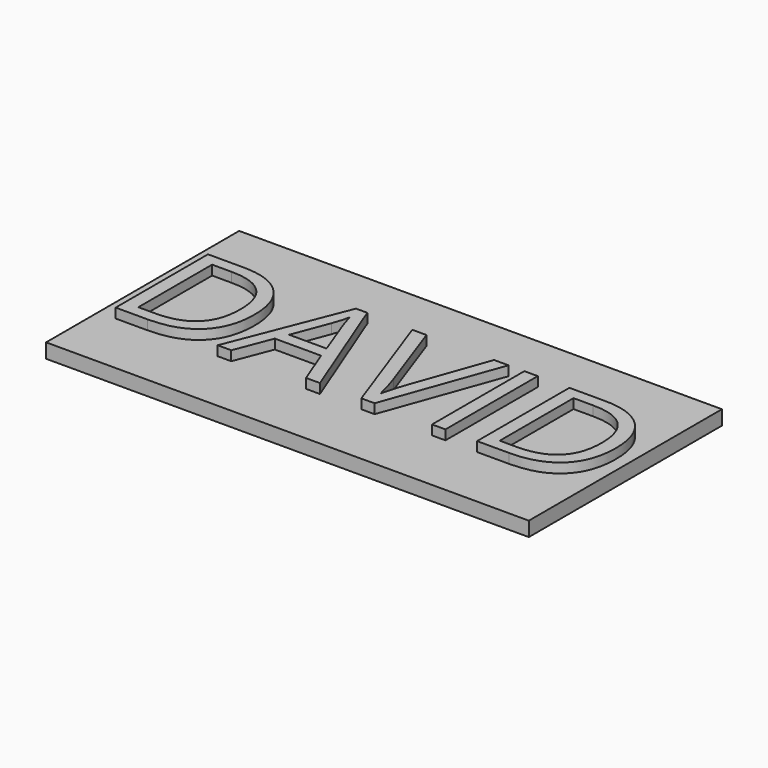
from build123d import *

# Parameters (mm, degrees)
F0_W         = 100
F0_H         = 50
F1_DEPTH     = 3
F2_TEXT_SIZE = 33.4849451772
F3_DEPTH     = 2


# Not quite as in the source:
# - Text() gives the source's letters only with a copy of the font that has no kerning and outlines rounded to 1/6400 em; it was checked with that copy


with BuildPart() as f1:
    # F0 (on Top) → F1 (new body)
    with BuildSketch(Plane.XY):
        Rectangle(F0_W, F0_H)
    extrude(amount=F1_DEPTH)

    # F2 (on face) → F3 (join)
    with BuildSketch(Plane.XY.offset(3)):
        with Locations((-49.7004427016, -11.4617320942)):
            Text('DAVID', F2_TEXT_SIZE, font='Open Sans', text_align=(TextAlign.LEFT, TextAlign.BOTTOM))
    extrude(amount=F3_DEPTH)


solid = f1.part
